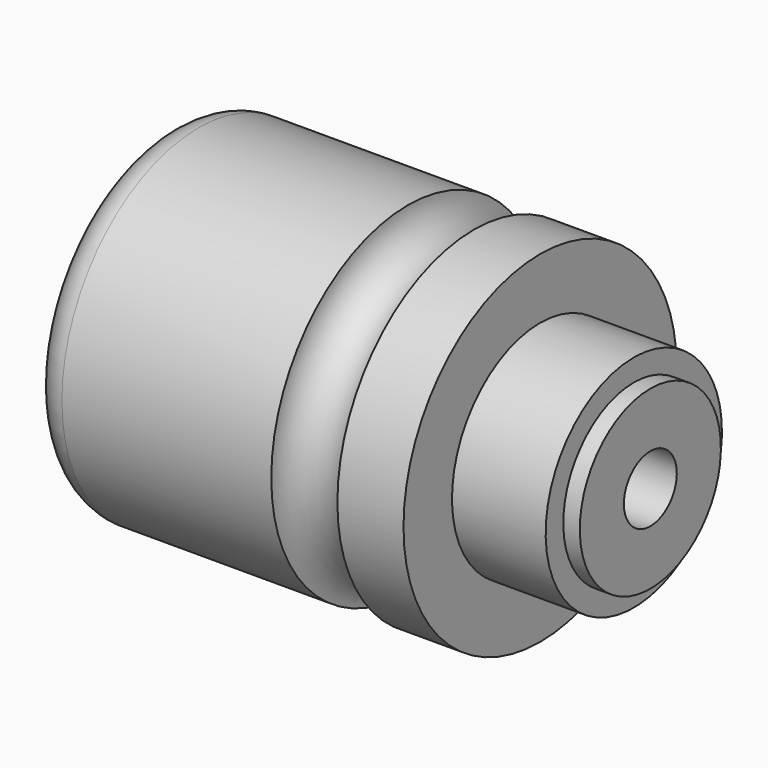
from build123d import *

# Parameters (mm, degrees)
F4_R = 5.99999


# Not quite as in the source:
# - a fillet or chamfer is up to 0.001 mm smaller than in the source, because OpenCascade refuses the exact size


with BuildPart() as f1:
    # F0 (on Front) → F1 (revolve)
    with BuildSketch(Plane.XZ):
        with BuildLine():
            Line((0, 31), (0, 0))
            Line((0, 0), (88, 0))
            Line((88, 0), (88, 16))
            Line((88, 16), (85, 16))
            Line((85, 16), (85, 20))
            Line((85, 20), (68, 20))
            Line((68, 20), (68, 31))
            Line((68, 31), (56, 31))
            ThreePointArc((56, 31), (50, 25), (44, 31))
            Line((44, 31), (0, 31))
        make_face()
    revolve(axis=Axis((44, 0, 0), (1, 0, 0)))

    # F2 (on Front) → F3 (revolve, cut)
    with BuildSketch(Plane.XZ):
        Polygon((0, 25), (0, 0), (88, 0), (88, 6), (30, 6), (30, 16), (22, 16), (22, 20.5), (15, 20.5), (15, 12.5), (12, 12.5), (12, 16), (1.5, 16), (1.5, 25), align=None)
    revolve(axis=Axis((44, 0, 0), (-1, 0, 0)), mode=Mode.SUBTRACT)

    # F4 (radius 6 in the source; OpenCascade refuses exactly that, so slightly less here)
    f4_edges = [f1.edges().sort_by_distance(p)[0] for p in [
        (0, 0, -31),
    ]]
    fillet(f4_edges, radius=F4_R)


solid = f1.part
